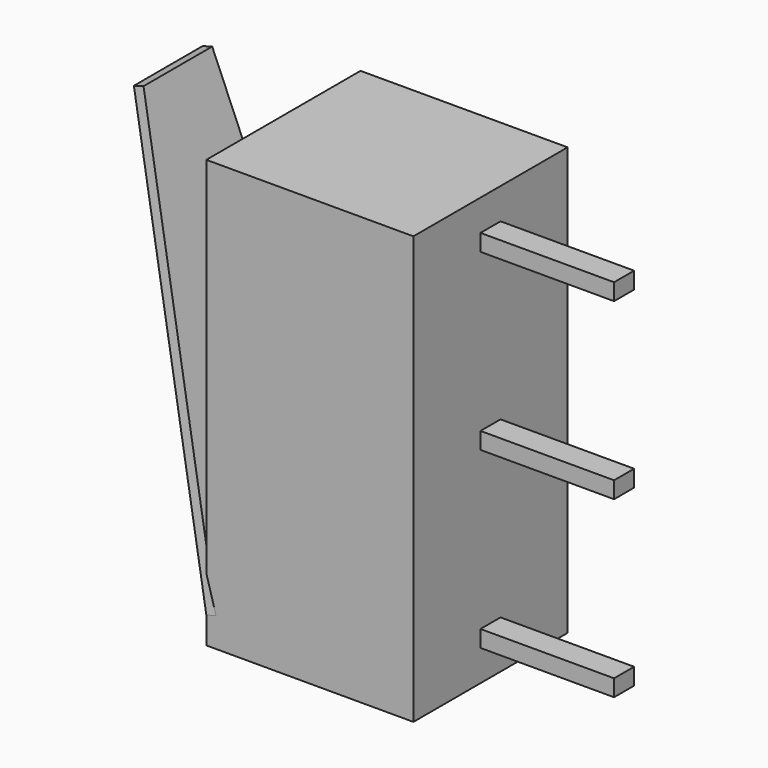
from build123d import *

# Parameters (mm, degrees)
F0_W     = 6.2
F0_H     = 12.8
F1_DEPTH = 5.77
F2_W     = 0.375
F2_H     = 0.5
F2_W_2   = 0.75
F3_DEPTH = 4
F6_W     = 5.77
F6_H     = 12.66
F7_DEPTH = 0.3
F9_DEPTH = 0.3


# Not quite as in the source:
# - the program builds the solid bodies; features that only make, move or delete a surface that nothing else refers to are left out


with BuildPart() as f1:
    # F0 (on Front) → F1 (new body)
    with BuildSketch(Plane.XZ):
        Rectangle(F0_W, F0_H)
    extrude(amount=F1_DEPTH)

    # F2 (on face) → F3 (join)
    with BuildSketch(Plane.YZ.offset(3.1)):
        with Locations((-2.6975, 5.22)):
            Rectangle(F2_W, F2_H)
        with Locations((-3.0725, 5.22)):
            Rectangle(F2_W, F2_H)
        with Locations((-2.885, 0)):
            Rectangle(F2_W_2, F2_H)
        with Locations((-3.0725, -5.22)):
            Rectangle(F2_W, F2_H)
        with Locations((-2.6975, -5.22)):
            Rectangle(F2_W, F2_H)
    extrude(amount=F3_DEPTH)

    # F6 (on face) → F7 (join)
    with BuildSketch(Plane(origin=(-4.3378860758, 0, -1.2283157987), x_dir=(0, -1, 0), z_dir=(-0.962170457, 0, -0.2724481816))):
        with Locations((2.885, 1.7864348038)):
            Rectangle(F6_W, F6_H)
    extrude(amount=-F7_DEPTH)

    # F8 (on face) → F9 (cut, through all)
    with BuildSketch(Plane(origin=(-4.3378860758, 0, -1.2283157987), x_dir=(0, -1, 0), z_dir=(-0.962170457, 0, -0.2724481816))):
        Polygon((0, -4.5435651962), (1.6, 8.1164348038), (0, 8.1164348038), align=None)
        Polygon((4.17, 8.1164348038), (5.77, -4.5435651962), (5.77, 8.1164348038), align=None)
    extrude(amount=-F9_DEPTH, mode=Mode.SUBTRACT)


solid = f1.part
